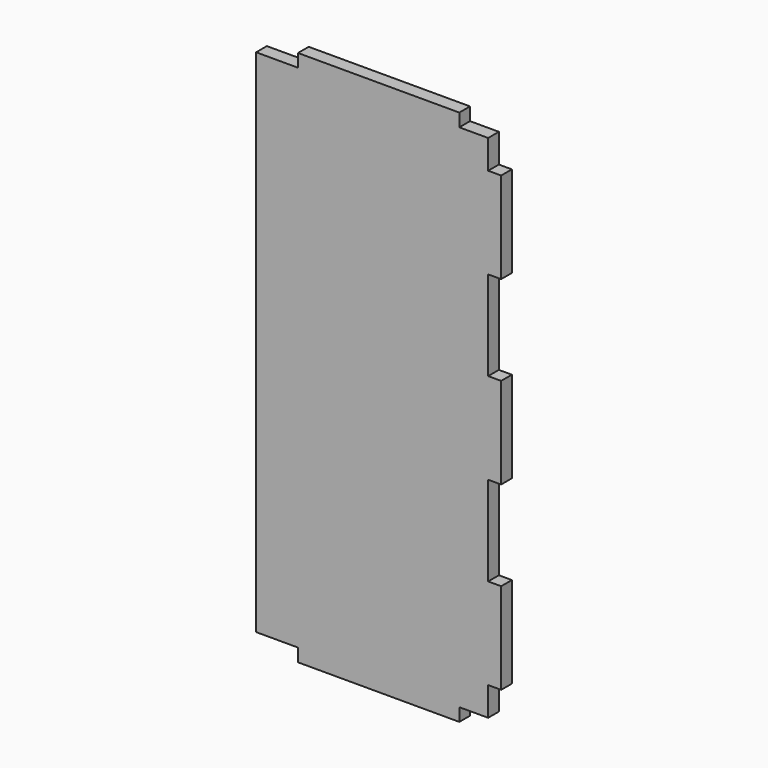
from build123d import *

# Parameters (mm, degrees)
F0_W     = 58
F0_H     = 127
F1_DEPTH = 3.175
F2_W     = 3.075
F2_H     = 21.2
F2_W_2   = 9.9
F2_H_2   = 3.075
F3_DEPTH = 25


# Not quite as in the source:
# - a length typed as a fraction of an inch, garbled in the dataset ("3 / 203.2 mm" for 3/8 in), is restored


with BuildPart() as f1:
    # F0 (on Front) → F1 (new body)
    with BuildSketch(Plane.XZ):
        Rectangle(F0_W, F0_H)
    extrude(amount=F1_DEPTH)

    # F2 (on face) → F3 (cut)
    with BuildSketch(Plane(origin=(0, 0, 0), x_dir=(-1, 0, 0), z_dir=(0, 1, 0))):
        Polygon((-19.1, 63.5), (-29, 63.5), (-29, 53.6), (-25.925, 53.6), (-25.925, 60.425), (-19.1, 60.425), align=None)
        with Locations((-27.4625, 21.4)):
            Rectangle(F2_W, F2_H)
        with Locations((-27.4625, -21.4)):
            Rectangle(F2_W, F2_H)
        Polygon((-25.925, -53.6), (-29, -53.6), (-29, -63.5), (-19.1, -63.5), (-19.1, -60.425), (-25.925, -60.425), align=None)
        with Locations((24.05, 61.9625)):
            Rectangle(F2_W_2, F2_H_2)
        with Locations((24.05, -61.9625)):
            Rectangle(F2_W_2, F2_H_2)
    extrude(amount=-F3_DEPTH, mode=Mode.SUBTRACT)


solid = f1.part
